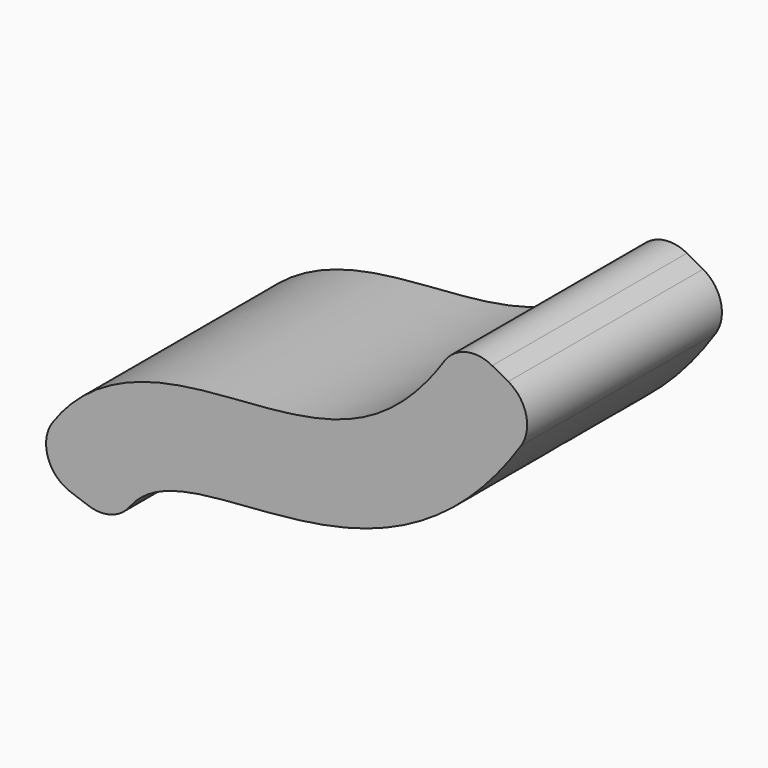
from build123d import *

# Parameters (mm, degrees)
F1_DEPTH = 50.8
F2_R     = 7.62


# Not quite as in the source:
# - the dataset's text gives a spline's control points without its knots; the knots are read off the source's solid


with BuildPart() as f1:
    # F0 (on Front) → F1 (new body)
    with BuildSketch(Plane.XZ):
        with BuildLine():
            Line((-55.0485830889, -7.3852598701), (-37.0773832593, -13.7049494734))
            add(Edge.make_bspline(
                [(-37.0773832593, -13.7049494734), (-27.6241134369, 13.1771620994), (20.1415180746, -20.9665218169), (51.3441984318, 35.9048443187)],
                knots=[0, 0, 0, 0, 101.3879073107, 101.3879073107, 101.3879073107, 101.3879073107], degree=3))
            Line((51.3441984318, 35.9048443187), (34.642799002, 45.0681274141))
            add(Edge.make_bspline(
                [(-55.0485830889, -7.3852598701), (-54.4926390919, -5.8043308542), (-53.1764213729, -2.6875146015), (-50.5314293038, 1.7278867732), (-47.2538632861, 5.6910743545), (-43.5082758092, 9.0216121231), (-39.5319485188, 11.6412421502), (-35.5389972848, 13.5945362808), (-31.6628107822, 15.0000075173), (-27.9581465021, 15.9916019071), (-24.4299846836, 16.6866792977), (-19.9382693628, 17.339586267), (-14.6614899569, 17.8227328201), (-8.7222195676, 18.2449955114), (-3.1169497995, 18.7421505919), (2.1567072949, 19.480252644), (7.091946379, 20.579587662), (11.7222503062, 22.1410595224), (16.1562527032, 24.2936211212), (20.5635300178, 27.2573066834), (25.0979351909, 31.3713560869), (29.8139291199, 37.0473286244), (33.0357743953, 42.1390942751), (34.642799002, 45.0681274141)],
                knots=[0, 0, 0, 0, 0.03125, 0.0625, 0.09375, 0.125, 0.15625, 0.1875, 0.21875, 0.25, 0.28125, 0.3125, 0.375, 0.4375, 0.5, 0.5625, 0.625, 0.6875, 0.75, 0.8125, 0.875, 0.9375, 1, 1, 1, 1], degree=3))
        make_face()
    extrude(amount=F1_DEPTH)

    # F2
    f2_edges = [f1.edges().sort_by_distance(p)[0] for p in [
        (34.642799, -25.4, 45.068127),
        (51.344198, -25.4, 35.904844),
        (-55.048583, -25.4, -7.38526),
        (-37.077383, -25.4, -13.704949),
    ]]
    fillet(f2_edges, radius=F2_R)


solid = f1.part
